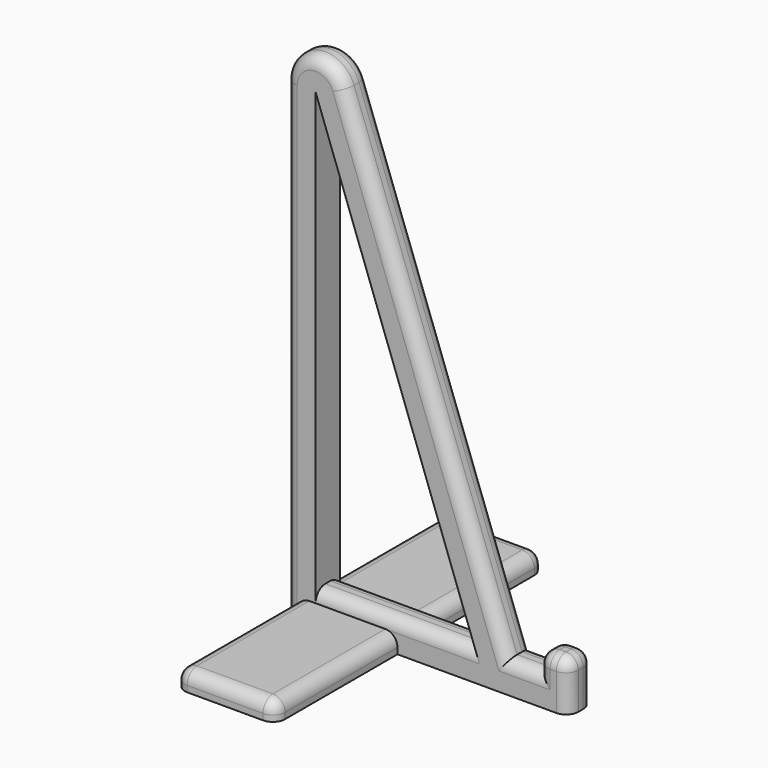
from build123d import *

# Parameters (mm, degrees)
F1_DEPTH    = 5
F3_W        = 10
F3_H        = 180
F4_DEPTH    = 5.001
F5_T1_DEPTH = 146.7820454904
F6_R        = 2
F11_DEPTH   = 25
F13_DEPTH   = 25
F14_R       = 2


# Not quite as in the source:
# - a fillet or chamfer that OpenCascade refuses, or shapes differently, is made with other operations: its cross-section is extruded or revolved along the edge and cut away or added
# - two fillets or chamfers of one size are made in one step


with BuildPart() as f1:
    # F0 (on Front) → F1 (new body)
    with BuildSketch(Plane.XZ):
        Polygon((-46.3970234266, 0), (0, 0), (0, 8), (-5, 8), (-5, 5), (-10, 5), (-46.3970234266, 105), align=None)
        Polygon((-41.3970234266, 5), (-41.3970234266, 76.6435909019), (-15.3208888624, 5), align=None, mode=Mode.SUBTRACT)
    extrude(amount=-F1_DEPTH)

    # F3 (on face) → F4 (cut, through all)
    with BuildSketch(Plane.XY.offset(5)):
        with Locations((-5, 95)):
            Rectangle(F3_W, F3_H)
    extrude(amount=-F4_DEPTH, mode=Mode.SUBTRACT)

    # F5: fillet of radius 5 on 1 edges, made by hand

    # F5_s2 → F5_t1 (cut)
    with BuildSketch(Plane.XZ.offset(-75.8910227452)):
        with BuildLine():
            ThreePointArc((-46.3970234266, 76.6435909019), (-42.265264315, 81.567629667), (-36.6985603227, 78.3536916185))
            Line((-36.6985603227, 78.3536916185), (-46.3970234266, 105))
            Line((-46.3970234266, 105), (-46.3970234266, 76.6435909019))
        make_face()
    extrude(amount=F5_T1_DEPTH, mode=Mode.SUBTRACT)

    # F6
    f6_edges = [f1.edges().sort_by_distance(p)[0] for p in [
        (-46.397023, 0, 38.321795),
        (-46.397023, 5, 38.321795),
        (-42.265264, 0, 81.56763),
        (-23.34928, 0, 41.676846),
        (-7.5, 0, 5),
        (-5, 0, 6.5),
        (-2.5, 0, 8),
        (0, 0, 4),
        (-28.358956, 0, 5),
        (-7.5, 5, 5),
        (-5, 5, 6.5),
        (-2.5, 5, 8),
        (0, 5, 4),
        (-42.265264, 5, 81.56763),
        (-23.34928, 5, 41.676846),
        (-28.358956, 5, 5),
        (-5, 2.5, 8),
        (0, 2.5, 8),
    ]]
    fillet(f6_edges, radius=F6_R)

    # F10 (on face) → F11 (join)
    with BuildSketch(Plane.XZ):
        Polygon((-44.3970234266, 3), (-44.3970234266, 0), (-27.9949859102, 0), (-27.9949859102, 3), (-41.3970234266, 3), align=None)
    extrude(amount=F11_DEPTH)

    # F12 (on face) → F13 (join)
    with BuildSketch(Plane(origin=(0, 5, 0), x_dir=(-1, 0, 0), z_dir=(0, 1, 0))):
        Polygon((27.9949859102, 0), (44.3970234266, 0), (44.3970234266, 3), (41.3970234266, 3), (27.9949859102, 3), align=None)
    extrude(amount=F13_DEPTH)

    # F14
    f14_edges = [f1.edges().sort_by_distance(p)[0] for p in [
        (-27.994986, -25, 1.5),
        (-44.397023, -25, 1.5),
        (-36.196005, -25, 3),
        (-27.994986, -12.5, 3),
        (-44.397023, -12.5, 3),
        (-27.994986, 30, 1.5),
        (-44.397023, 30, 1.5),
        (-27.994986, 17.5, 3),
        (-36.196005, 30, 3),
        (-44.397023, 17.5, 3),
    ]]
    fillet(f14_edges, radius=F14_R)


solid = f1.part
